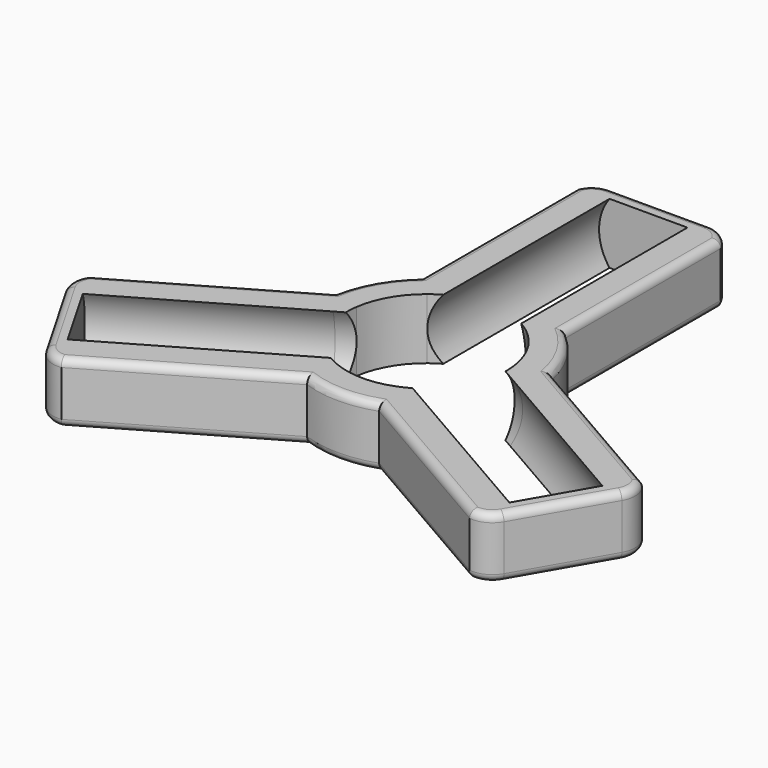
from build123d import *

# Parameters (mm, degrees)
F1_DEPTH       = 4
F3_R           = 6.5
F6_R           = 6.5
F9_R           = 6.5
F11_DEPTH      = 4
F12_T1_DEPTH   = 13
F12_T3_DEPTH   = 13
F12_T5_DEPTH   = 13
F12_T10_DEPTH  = 30.5455488499
F12_S11_R      = 14.5
F12_T12_DEPTH  = 17
F12_T16_DEPTH  = 30.5455488499
F12_S17_R      = 14.5
F12_T18_DEPTH  = 17
F12_T22_ANGLE  = 57.8931407827
F12_T28_DEPTH  = 30.5455488499
F12_S29_R      = 14.5
F12_T30_DEPTH  = 17
F12_T34_DEPTH  = 30.5455488499
F12_S35_R      = 14.5
F12_T36_DEPTH  = 17
F12_T40_ANGLE  = 57.8931407827
F12_T46_DEPTH  = 30.5455488499
F12_S47_R      = 14.5
F12_T48_DEPTH  = 17
F12_T52_DEPTH  = 30.5455488499
F12_S53_R      = 14.5
F12_T54_DEPTH  = 17
F12_T58_ANGLE  = 57.8931407827
F12_T64_DEPTH  = 30.5455488499
F12_S65_R      = 14.5
F12_T66_DEPTH  = 17
F12_T70_ANGLE  = 57.8931407827
F12_T76_DEPTH  = 30.5455488499
F12_S77_R      = 14.5
F12_T78_DEPTH  = 17
F12_T82_DEPTH  = 30.5455488499
F12_S83_R      = 14.5
F12_T84_DEPTH  = 17
F12_T88_ANGLE  = 57.8931407827
F12_T94_DEPTH  = 30.5455488499
F12_S95_R      = 14.5
F12_T96_DEPTH  = 17
F12_T100_DEPTH = 30.5455488499
F12_S101_R     = 14.5
F12_T102_DEPTH = 17
F12_T106_ANGLE = 57.8931407827
F12_T112_DEPTH = 30.5455488499
F12_S113_R     = 14.5
F12_T114_DEPTH = 17
F12_T116_ANGLE = 111.4637339609
F12_T118_ANGLE = 111.4637339609
F12_T120_ANGLE = 111.4637339609
F12_T122_ANGLE = 111.4637339609
F12_T124_ANGLE = 111.4637339609
F12_T126_ANGLE = 111.4637339609
F12_T128_ANGLE = 111.4637339609
F12_T130_ANGLE = 111.4637339609
F12_T132_ANGLE = 111.4637339609
F12_T134_ANGLE = 111.4637339609
F12_T136_ANGLE = 111.4637339609
F12_T138_ANGLE = 111.4637339609
F12_T143_DEPTH = 30.5455488499
F12_S144_R     = 14.5
F12_T145_DEPTH = 17
F12_T148_ANGLE = 57.8931407827
F12_T155_ANGLE = 57.8931407827
F12_T159_DEPTH = 30.5455488499
F12_S160_R     = 14.5
F12_T161_DEPTH = 17
F12_T167_DEPTH = 30.5455488499
F12_S168_R     = 14.5
F12_T169_DEPTH = 17
F12_T172_ANGLE = 57.8931407827
F12_T179_DEPTH = 30.5455488499
F12_S180_R     = 14.5
F12_T181_DEPTH = 17
F12_T184_ANGLE = 57.8931407827
F12_T191_ANGLE = 57.8931407827
F12_T195_DEPTH = 30.5455488499
F12_S196_R     = 14.5
F12_T197_DEPTH = 17
F12_T203_DEPTH = 30.5455488499
F12_S204_R     = 14.5
F12_T205_DEPTH = 17
F12_T208_ANGLE = 57.8931407827
F12_T215_ANGLE = 57.8931407827
F12_T219_DEPTH = 30.5455488499
F12_S220_R     = 14.5
F12_T221_DEPTH = 17
F12_T227_DEPTH = 30.5455488499
F12_S228_R     = 14.5
F12_T229_DEPTH = 17
F12_T232_ANGLE = 57.8931407827
F12_T239_ANGLE = 57.8931407827
F12_T243_DEPTH = 30.5455488499
F12_S244_R     = 14.5
F12_T245_DEPTH = 17
F12_T251_DEPTH = 30.5455488499
F12_S252_R     = 14.5
F12_T253_DEPTH = 17
F12_T256_ANGLE = 57.8931407827
F12_T263_ANGLE = 57.8931407827
F12_T267_DEPTH = 30.5455488499
F12_S268_R     = 14.5
F12_T269_DEPTH = 17
F12_T275_DEPTH = 30.5455488499
F12_S276_R     = 14.5
F12_T277_DEPTH = 17
F12_T280_ANGLE = 57.8931407827


# Not quite as in the source:
# - a fillet or chamfer that OpenCascade refuses, or shapes differently, is made with other operations: its cross-section is extruded or revolved along the edge and cut away or added


with BuildPart() as f1:
    # F0 (on Top) → F1 (new body, symmetric)
    with BuildSketch(Plane.XY):
        with BuildLine():
            ThreePointArc((-9.5, 10.9544511501), (-8.0626945002, 12.0516786133), (-6.5, 12.9614813968))
            Line((-6.5, 12.9614813968), (-6.5, 36.5))
            Line((-6.5, 36.5), (-9.5, 36.5))
            Line((-9.5, 36.5), (-9.5, 10.9544511501))
        make_face()
        with BuildLine():
            Line((6.5, 36.5), (6.5, 12.9614813968))
            ThreePointArc((6.5, 12.9614813968), (8.0626945002, 12.0516786133), (9.5, 10.9544511501))
            Line((9.5, 10.9544511501), (9.5, 36.5))
            Line((9.5, 36.5), (6.5, 36.5))
        make_face()
        with BuildLine():
            ThreePointArc((0, 10.5), (3.4398242587, 9.9205649571), (6.5, 8.2462112512))
            Line((6.5, 8.2462112512), (6.5, 12.9614813968))
            ThreePointArc((6.5, 12.9614813968), (3.3397993762, 14.1101289904), (0, 14.5))
            Line((0, 14.5), (0, 10.5))
        make_face()
        with BuildLine():
            ThreePointArc((6.5, 8.2462112512), (9.0932667397, 5.25), (10.3914284285, 1.506059499))
            Line((10.3914284285, 1.506059499), (14.4749721603, -0.8515755738))
            ThreePointArc((14.4749721603, -0.8515755738), (14.4937416895, -0.4259716395), (14.5, 0))
            ThreePointArc((14.5, 0), (14.4340583035, 1.3812895755), (14.2368329805, 2.7500157609))
            ThreePointArc((14.2368329805, 2.7500157609), (12.5573683549, 7.25), (9.5, 10.9544511501))
            ThreePointArc((9.5, 10.9544511501), (8.0626945002, 12.0516786133), (6.5, 12.9614813968))
            Line((6.5, 12.9614813968), (6.5, 8.2462112512))
        make_face()
        with BuildLine():
            ThreePointArc((-6.5, 8.2462112512), (-3.4398242587, 9.9205649571), (0, 10.5))
            Line((0, 10.5), (0, 14.5))
            ThreePointArc((0, 14.5), (-3.3397993762, 14.1101289904), (-6.5, 12.9614813968))
            Line((-6.5, 12.9614813968), (-6.5, 8.2462112512))
        make_face()
        with BuildLine():
            ThreePointArc((-10.3914284285, 1.506059499), (-9.0932667397, 5.25), (-6.5, 8.2462112512))
            Line((-6.5, 8.2462112512), (-6.5, 12.9614813968))
            ThreePointArc((-6.5, 12.9614813968), (-8.0626945002, 12.0516786133), (-9.5, 10.9544511501))
            ThreePointArc((-9.5, 10.9544511501), (-12.5573683549, 7.25), (-14.2368329805, 2.7500157609))
            ThreePointArc((-14.2368329805, 2.7500157609), (-14.4684070874, 0.9566589535), (-14.4749721603, -0.8515755738))
            Line((-14.4749721603, -0.8515755738), (-10.3914284285, 1.506059499))
        make_face()
        with BuildLine():
            Line((-34.8599272381, -12.6208348754), (-14.4749721603, -0.8515755738))
            ThreePointArc((-14.4749721603, -0.8515755738), (-14.4684070874, 0.9566589535), (-14.2368329805, 2.7500157609))
            Line((-14.2368329805, 2.7500157609), (-36.3599272381, -10.022758664))
            Line((-36.3599272381, -10.022758664), (-34.8599272381, -12.6208348754))
        make_face()
        with BuildLine():
            Line((-12.5573683549, -7.25), (-9.0932667397, -5.25))
            ThreePointArc((-9.0932667397, -5.25), (-10.3113734022, -1.981307286), (-10.3914284285, 1.506059499))
            Line((-10.3914284285, 1.506059499), (-14.4749721603, -0.8515755738))
            ThreePointArc((-14.4749721603, -0.8515755738), (-13.8896298445, -4.1627133919), (-12.5573683549, -7.25))
        make_face()
        with BuildLine():
            Line((-7.9749721603, -12.109905823), (-3.8914284285, -9.7522707502))
            ThreePointArc((-3.8914284285, -9.7522707502), (-6.8715491434, -7.9392576712), (-9.0932667397, -5.25))
            Line((-9.0932667397, -5.25), (-12.5573683549, -7.25))
            ThreePointArc((-12.5573683549, -7.25), (-10.5498304683, -9.9474155985), (-7.9749721603, -12.109905823))
        make_face()
        with BuildLine():
            ThreePointArc((-4.7368329805, -13.704466911), (-6.4057125872, -13.0083375667), (-7.9749721603, -12.109905823))
            Line((-7.9749721603, -12.109905823), (-28.3599272381, -23.8791651246))
            Line((-28.3599272381, -23.8791651246), (-26.8599272381, -26.477241336))
            Line((-26.8599272381, -26.477241336), (-4.7368329805, -13.704466911))
        make_face()
        with BuildLine():
            Line((7.9749721603, -12.109905823), (3.8914284285, -9.7522707502))
            ThreePointArc((3.8914284285, -9.7522707502), (0, -10.5), (-3.8914284285, -9.7522707502))
            Line((-3.8914284285, -9.7522707502), (-7.9749721603, -12.109905823))
            ThreePointArc((-7.9749721603, -12.109905823), (-6.4057125872, -13.0083375667), (-4.7368329805, -13.704466911))
            ThreePointArc((-4.7368329805, -13.704466911), (0, -14.5), (4.7368329805, -13.704466911))
            ThreePointArc((4.7368329805, -13.704466911), (6.4057125872, -13.0083375667), (7.9749721603, -12.109905823))
        make_face()
        with BuildLine():
            Line((28.3599272381, -23.8791651246), (7.9749721603, -12.109905823))
            ThreePointArc((7.9749721603, -12.109905823), (6.4057125872, -13.0083375667), (4.7368329805, -13.704466911))
            Line((4.7368329805, -13.704466911), (26.8599272381, -26.477241336))
            Line((26.8599272381, -26.477241336), (28.3599272381, -23.8791651246))
        make_face()
        with BuildLine():
            Line((12.5573683549, -7.25), (9.0932667397, -5.25))
            ThreePointArc((9.0932667397, -5.25), (6.8715491434, -7.9392576712), (3.8914284285, -9.7522707502))
            Line((3.8914284285, -9.7522707502), (7.9749721603, -12.109905823))
            ThreePointArc((7.9749721603, -12.109905823), (10.5498304683, -9.9474155985), (12.5573683549, -7.25))
        make_face()
        with BuildLine():
            ThreePointArc((10.3914284285, 1.506059499), (10.4728219335, 0.7549839403), (10.5, 0))
            ThreePointArc((10.5, 0), (10.142221176, -2.7175999736), (9.0932667397, -5.25))
            Line((9.0932667397, -5.25), (12.5573683549, -7.25))
            ThreePointArc((12.5573683549, -7.25), (13.8896298445, -4.1627133919), (14.4749721603, -0.8515755738))
            Line((14.4749721603, -0.8515755738), (10.3914284285, 1.506059499))
        make_face()
        with BuildLine():
            ThreePointArc((14.5, 0), (14.4937416895, -0.4259716395), (14.4749721603, -0.8515755738))
            Line((14.4749721603, -0.8515755738), (34.8599272381, -12.6208348754))
            Line((34.8599272381, -12.6208348754), (36.3599272381, -10.022758664))
            Line((36.3599272381, -10.022758664), (14.2368329805, 2.7500157609))
            ThreePointArc((14.2368329805, 2.7500157609), (14.4340583035, 1.3812895755), (14.5, 0))
        make_face()
        with BuildLine():
            ThreePointArc((0, 14.5), (3.3397993762, 14.1101289904), (6.5, 12.9614813968))
            Line((6.5, 12.9614813968), (6.5, 36.5))
            Line((6.5, 36.5), (0, 36.5))
            Line((0, 36.5), (0, 14.5))
        make_face()
        with BuildLine():
            ThreePointArc((-6.5, 12.9614813968), (-3.3397993762, 14.1101289904), (0, 14.5))
            Line((0, 14.5), (0, 36.5))
            Line((0, 36.5), (-6.5, 36.5))
            Line((-6.5, 36.5), (-6.5, 12.9614813968))
        make_face()
        with BuildLine():
            Line((-31.6099272381, -18.25), (-12.5573683549, -7.25))
            ThreePointArc((-12.5573683549, -7.25), (-13.8896298445, -4.1627133919), (-14.4749721603, -0.8515755738))
            Line((-14.4749721603, -0.8515755738), (-34.8599272381, -12.6208348754))
            Line((-34.8599272381, -12.6208348754), (-31.6099272381, -18.25))
        make_face()
        with BuildLine():
            Line((-28.3599272381, -23.8791651246), (-7.9749721603, -12.109905823))
            ThreePointArc((-7.9749721603, -12.109905823), (-10.5498304683, -9.9474155985), (-12.5573683549, -7.25))
            Line((-12.5573683549, -7.25), (-31.6099272381, -18.25))
            Line((-31.6099272381, -18.25), (-28.3599272381, -23.8791651246))
        make_face()
        with BuildLine():
            Line((31.6099272381, -18.25), (12.5573683549, -7.25))
            ThreePointArc((12.5573683549, -7.25), (10.5498304683, -9.9474155985), (7.9749721603, -12.109905823))
            Line((7.9749721603, -12.109905823), (28.3599272381, -23.8791651246))
            Line((28.3599272381, -23.8791651246), (31.6099272381, -18.25))
        make_face()
        with BuildLine():
            Line((34.8599272381, -12.6208348754), (14.4749721603, -0.8515755738))
            ThreePointArc((14.4749721603, -0.8515755738), (13.8896298445, -4.1627133919), (12.5573683549, -7.25))
            Line((12.5573683549, -7.25), (31.6099272381, -18.25))
            Line((31.6099272381, -18.25), (34.8599272381, -12.6208348754))
        make_face()
    extrude(amount=F1_DEPTH, both=True)

    # F4: sweep along a path in F0
    with BuildLine(Plane.XY) as f4_path:
        Line((0, 36.5), (0, 10.5))
        Line((0, 10.5), (0, 5.0456705503))
    # F3 (on offset) → F4 (sweep, cut)
    with BuildSketch(Plane(origin=(0, 36.5, 0), x_dir=(-1, 0, 0), z_dir=(0, 1, 0))):
        Circle(F3_R)
    sweep(path=f4_path.line, mode=Mode.SUBTRACT)

    # F7: sweep along a path in F0
    with BuildLine(Plane.XY) as f7_path:
        Line((-31.6099272381, -18.25), (-9.0932667397, -5.25))
        Line((-9.0932667397, -5.25), (-4.3696788757, -2.5228352752))
    # F6 (on offset) → F7 (sweep, cut)
    with BuildSketch(Plane(origin=(-31.6099272381, -18.25, 0), x_dir=(0.5, -0.8660254038, 0), z_dir=(-0.8660254038, -0.5, 0))):
        Circle(F6_R)
    sweep(path=f7_path.line, mode=Mode.SUBTRACT)

    # F10: sweep along a path in F0
    with BuildLine(Plane.XY) as f10_path:
        Line((31.6099272381, -18.25), (9.0932667397, -5.25))
        Line((9.0932667397, -5.25), (4.3696788757, -2.5228352752))
    # F9 (on offset) → F10 (sweep, cut)
    with BuildSketch(Plane(origin=(31.6099272381, -18.25, 0), x_dir=(0.5, 0.8660254038, 0), z_dir=(0.8660254038, -0.5, 0))):
        Circle(F9_R)
    sweep(path=f10_path.line, mode=Mode.SUBTRACT)

    # F0 (on Top) → F11 (join, symmetric)
    with BuildSketch(Plane.XY):
        with BuildLine():
            Line((0, 36.5), (6.5, 36.5))
            Line((6.5, 36.5), (9.5, 36.5))
            ThreePointArc((9.5, 36.5), (8.3027756377, 37.9541634566), (6.5, 38.5))
            Line((6.5, 38.5), (0, 38.5))
            Line((0, 38.5), (-6.5, 38.5))
            ThreePointArc((-6.5, 38.5), (-8.3027756377, 37.9541634566), (-9.5, 36.5))
            Line((-9.5, 36.5), (-6.5, 36.5))
            Line((-6.5, 36.5), (0, 36.5))
        make_face()
        with BuildLine():
            Line((-26.8599272381, -26.477241336), (-28.3599272381, -23.8791651246))
            Line((-28.3599272381, -23.8791651246), (-31.6099272381, -18.25))
            Line((-31.6099272381, -18.25), (-34.8599272381, -12.6208348754))
            Line((-34.8599272381, -12.6208348754), (-36.3599272381, -10.022758664))
            ThreePointArc((-36.3599272381, -10.022758664), (-37.0206575517, -11.7866671041), (-36.5919780457, -13.6208348754))
            Line((-36.5919780457, -13.6208348754), (-33.3419780457, -19.25))
            Line((-33.3419780457, -19.25), (-30.0919780457, -24.8791651246))
            ThreePointArc((-30.0919780457, -24.8791651246), (-28.7178819139, -26.1674963525), (-26.8599272381, -26.477241336))
        make_face()
        with BuildLine():
            Line((36.3599272381, -10.022758664), (34.8599272381, -12.6208348754))
            Line((34.8599272381, -12.6208348754), (31.6099272381, -18.25))
            Line((31.6099272381, -18.25), (28.3599272381, -23.8791651246))
            Line((28.3599272381, -23.8791651246), (26.8599272381, -26.477241336))
            ThreePointArc((26.8599272381, -26.477241336), (28.7178819139, -26.1674963525), (30.0919780457, -24.8791651246))
            Line((30.0919780457, -24.8791651246), (33.3419780457, -19.25))
            Line((33.3419780457, -19.25), (36.5919780457, -13.6208348754))
            ThreePointArc((36.5919780457, -13.6208348754), (37.0206575517, -11.7866671041), (36.3599272381, -10.022758664))
        make_face()
    extrude(amount=F11_DEPTH, both=True)

    # F12: fillet of radius 1 on 24 edges, made by hand

    # F12_s2 → F12_t1 (cut)
    with BuildSketch(Plane.YZ.offset(-6.5)):
        with BuildLine():
            ThreePointArc((37.5, -4), (38.2071067812, -3.7071067812), (38.5, -3))
            Line((38.5, -3), (38.5, -4))
            Line((38.5, -4), (37.5, -4))
        make_face()
        with BuildLine():
            ThreePointArc((37.5, 4), (38.2071067812, 3.7071067812), (38.5, 3))
            Line((38.5, 3), (38.5, 4))
            Line((38.5, 4), (37.5, 4))
        make_face()
    extrude(amount=F12_T1_DEPTH, mode=Mode.SUBTRACT)

    # F12_s4 → F12_t3 (cut)
    with BuildSketch(Plane(origin=(-3.25, 5.6291651246, 0), x_dir=(0, 0, 1), z_dir=(0.5, -0.8660254038, 0))):
        with BuildLine():
            ThreePointArc((-4, 37.5), (-3.7071067812, 38.2071067812), (-3, 38.5))
            Line((-3, 38.5), (-4, 38.5))
            Line((-4, 38.5), (-4, 37.5))
        make_face()
        with BuildLine():
            ThreePointArc((4, 37.5), (3.7071067812, 38.2071067812), (3, 38.5))
            Line((3, 38.5), (4, 38.5))
            Line((4, 38.5), (4, 37.5))
        make_face()
    extrude(amount=F12_T3_DEPTH, mode=Mode.SUBTRACT)

    # F12_s6 → F12_t5 (cut)
    with BuildSketch(Plane(origin=(-3.25, -5.6291651246, 0), x_dir=(0, 0, 1), z_dir=(0.5, 0.8660254038, 0))):
        with BuildLine():
            ThreePointArc((-4, 37.5), (-3.7071067812, 38.2071067812), (-3, 38.5))
            Line((-3, 38.5), (-4, 38.5))
            Line((-4, 38.5), (-4, 37.5))
        make_face()
        with BuildLine():
            ThreePointArc((4, 37.5), (3.7071067812, 38.2071067812), (3, 38.5))
            Line((3, 38.5), (4, 38.5))
            Line((4, 38.5), (4, 37.5))
        make_face()
    extrude(amount=F12_T5_DEPTH, mode=Mode.SUBTRACT)


with BuildPart() as f12_tool8:
    # F12_s9 → F12_t10 (new body)
    with BuildSketch(Plane.XZ.offset(-39)):
        with BuildLine():
            ThreePointArc((-9.5, -3), (-9.2071067812, -3.7071067812), (-8.5, -4))
            Line((-8.5, -4), (-9.5, -4))
            Line((-9.5, -4), (-9.5, -3))
        make_face()
    extrude(amount=F12_T10_DEPTH)

    # F12_s11 → F12_t12 (cut, symmetric)
    with BuildSketch(Plane.XY.offset(-3.5)):
        Circle(F12_S11_R)
    extrude(amount=F12_T12_DEPTH, both=True, mode=Mode.SUBTRACT)


with BuildPart() as f1_1:
    add(f1.part)

    # F12_t7: cut F12_tool8
    add(f12_tool8.part, mode=Mode.SUBTRACT)


with BuildPart() as f12_tool14:
    # F12_s15 → F12_t16 (new body)
    with BuildSketch(Plane.XZ.offset(-8.4544511501)):
        with BuildLine():
            ThreePointArc((8.5, -4), (9.2071067812, -3.7071067812), (9.5, -3))
            Line((9.5, -3), (9.5, -4))
            Line((9.5, -4), (8.5, -4))
        make_face()
    extrude(amount=-F12_T16_DEPTH)

    # F12_s17 → F12_t18 (cut, symmetric)
    with BuildSketch(Plane.XY.offset(-3.5)):
        Circle(F12_S17_R)
    extrude(amount=F12_T18_DEPTH, both=True, mode=Mode.SUBTRACT)


with BuildPart() as f1_2:
    add(f1_1.part)

    # F12_t13: cut F12_tool14
    add(f12_tool14.part, mode=Mode.SUBTRACT)


with BuildPart() as f12_tool20:
    # F12_s21 → F12_t22 (revolve)
    with BuildSketch(Plane(origin=(0, 0, 0), x_dir=(0, 0, 1), z_dir=(0.8566866434, 0.5158371787, 0))):
        with BuildLine():
            ThreePointArc((-4, -13.5), (-3.7071067812, -14.2071067812), (-3, -14.5))
            Line((-3, -14.5), (-4, -14.5))
            Line((-4, -14.5), (-4, -13.5))
        make_face()
    revolve(axis=Axis((0, 0, -4), (0, 0, 1)), revolution_arc=F12_T22_ANGLE)

    split(bisect_by=Plane.YZ.offset(-9.5), keep=Keep.BOTTOM)

    split(bisect_by=Plane(origin=(-4.75, 8.227241336, 0), x_dir=(0, 0, 1), z_dir=(-0.5, 0.8660254038, 0)), keep=Keep.TOP)


with BuildPart() as f1_3:
    add(f1_2.part)

    # F12_t19: cut F12_tool20
    add(f12_tool20.part, mode=Mode.SUBTRACT)


with BuildPart() as f12_tool26:
    # F12_s27 → F12_t28 (new body)
    with BuildSketch(Plane(origin=(-7.321769471, -4.2272255751, 0), x_dir=(0, 0, 1), z_dir=(-0.8660254038, -0.5, 0))):
        with BuildLine():
            ThreePointArc((-4, 8.5), (-3.7071067812, 9.2071067812), (-3, 9.5))
            Line((-3, 9.5), (-4, 9.5))
            Line((-4, 9.5), (-4, 8.5))
        make_face()
    extrude(amount=F12_T28_DEPTH)

    # F12_s29 → F12_t30 (cut, symmetric)
    with BuildSketch(Plane.XY.offset(-3.5)):
        Circle(F12_S29_R)
    extrude(amount=F12_T30_DEPTH, both=True, mode=Mode.SUBTRACT)


with BuildPart() as f1_4:
    add(f1_3.part)

    # F12_t25: cut F12_tool26
    add(f12_tool26.part, mode=Mode.SUBTRACT)


with BuildPart() as f12_tool32:
    # F12_s33 → F12_t34 (new body)
    with BuildSketch(Plane(origin=(-33.7749907476, -19.5, 0), x_dir=(0, 0, 1), z_dir=(0.8660254038, 0.5, 0))):
        with BuildLine():
            ThreePointArc((-4, 8.5), (-3.7071067812, 9.2071067812), (-3, 9.5))
            Line((-3, 9.5), (-4, 9.5))
            Line((-4, 9.5), (-4, 8.5))
        make_face()
    extrude(amount=F12_T34_DEPTH)

    # F12_s35 → F12_t36 (cut, symmetric)
    with BuildSketch(Plane.XY.offset(-3.5)):
        Circle(F12_S35_R)
    extrude(amount=F12_T36_DEPTH, both=True, mode=Mode.SUBTRACT)


with BuildPart() as f1_5:
    add(f1_4.part)

    # F12_t31: cut F12_tool32
    add(f12_tool32.part, mode=Mode.SUBTRACT)


with BuildPart() as f12_tool38:
    # F12_s39 → F12_t40 (revolve)
    with BuildSketch(Plane(origin=(0, 0, 0), x_dir=(0, 0, 1), z_dir=(-0.8750714227, 0.4839938069, 0))):
        with BuildLine():
            ThreePointArc((-4, -13.5), (-3.7071067812, -14.2071067812), (-3, -14.5))
            Line((-3, -14.5), (-4, -14.5))
            Line((-4, -14.5), (-4, -13.5))
        make_face()
    revolve(axis=Axis((0, 0, -4), (0, 0, 1)), revolution_arc=F12_T40_ANGLE)

    split(bisect_by=Plane(origin=(-4.75, -8.227241336, 0), x_dir=(0, 0, 1), z_dir=(-0.5, -0.8660254038, 0)), keep=Keep.TOP)

    split(bisect_by=Plane(origin=(4.75, -8.227241336, 0), x_dir=(0, 0, 1), z_dir=(0.5, -0.8660254038, 0)), keep=Keep.TOP)


with BuildPart() as f1_6:
    add(f1_5.part)

    # F12_t37: cut F12_tool38
    add(f12_tool38.part, mode=Mode.SUBTRACT)


with BuildPart() as f12_tool44:
    # F12_s45 → F12_t46 (new body)
    with BuildSketch(Plane(origin=(7.321769471, -4.2272255751, 0), x_dir=(0, 0, 1), z_dir=(0.8660254038, -0.5, 0))):
        with BuildLine():
            ThreePointArc((-4, 8.5), (-3.7071067812, 9.2071067812), (-3, 9.5))
            Line((-3, 9.5), (-4, 9.5))
            Line((-4, 9.5), (-4, 8.5))
        make_face()
    extrude(amount=F12_T46_DEPTH)

    # F12_s47 → F12_t48 (cut, symmetric)
    with BuildSketch(Plane.XY.offset(-3.5)):
        Circle(F12_S47_R)
    extrude(amount=F12_T48_DEPTH, both=True, mode=Mode.SUBTRACT)


with BuildPart() as f1_7:
    add(f1_6.part)

    # F12_t43: cut F12_tool44
    add(f12_tool44.part, mode=Mode.SUBTRACT)


with BuildPart() as f12_tool50:
    # F12_s51 → F12_t52 (new body)
    with BuildSketch(Plane(origin=(33.7749907476, -19.5, 0), x_dir=(0, 0, 1), z_dir=(-0.8660254038, 0.5, 0))):
        with BuildLine():
            ThreePointArc((-4, 8.5), (-3.7071067812, 9.2071067812), (-3, 9.5))
            Line((-3, 9.5), (-4, 9.5))
            Line((-4, 9.5), (-4, 8.5))
        make_face()
    extrude(amount=F12_T52_DEPTH)

    # F12_s53 → F12_t54 (cut, symmetric)
    with BuildSketch(Plane.XY.offset(-3.5)):
        Circle(F12_S53_R)
    extrude(amount=F12_T54_DEPTH, both=True, mode=Mode.SUBTRACT)


with BuildPart() as f1_8:
    add(f1_7.part)

    # F12_t49: cut F12_tool50
    add(f12_tool50.part, mode=Mode.SUBTRACT)


with BuildPart() as f12_tool56:
    # F12_s57 → F12_t58 (revolve)
    with BuildSketch(Plane(origin=(0, 0, 0), x_dir=(0, 0, 1), z_dir=(0.0183847793, -0.9998309857, 0))):
        with BuildLine():
            ThreePointArc((-4, -13.5), (-3.7071067812, -14.2071067812), (-3, -14.5))
            Line((-3, -14.5), (-4, -14.5))
            Line((-4, -14.5), (-4, -13.5))
        make_face()
    revolve(axis=Axis((0, 0, -4), (0, 0, 1)), revolution_arc=F12_T58_ANGLE)

    split(bisect_by=Plane.YZ.offset(9.5), keep=Keep.TOP)

    split(bisect_by=Plane(origin=(4.75, 8.227241336, 0), x_dir=(0, 0, 1), z_dir=(0.5, 0.8660254038, 0)), keep=Keep.TOP)


with BuildPart() as f1_9:
    add(f1_8.part)

    # F12_t55: cut F12_tool56
    add(f12_tool56.part, mode=Mode.SUBTRACT)


with BuildPart() as f12_tool62:
    # F12_s63 → F12_t64 (new body)
    with BuildSketch(Plane.XZ.offset(-8.4544511501)):
        with BuildLine():
            ThreePointArc((8.5, 4), (9.2071067812, 3.7071067812), (9.5, 3))
            Line((9.5, 3), (9.5, 4))
            Line((9.5, 4), (8.5, 4))
        make_face()
    extrude(amount=-F12_T64_DEPTH)

    # F12_s65 → F12_t66 (cut, symmetric)
    with BuildSketch(Plane.XY.offset(3.5)):
        Circle(F12_S65_R)
    extrude(amount=F12_T66_DEPTH, both=True, mode=Mode.SUBTRACT)


with BuildPart() as f1_10:
    add(f1_9.part)

    # F12_t61: cut F12_tool62
    add(f12_tool62.part, mode=Mode.SUBTRACT)


with BuildPart() as f12_tool68:
    # F12_s69 → F12_t70 (revolve)
    with BuildSketch(Plane(origin=(0, 0, 0), x_dir=(0, 0, 1), z_dir=(0.0183847793, -0.9998309857, 0))):
        with BuildLine():
            ThreePointArc((4, -13.5), (3.7071067812, -14.2071067812), (3, -14.5))
            Line((3, -14.5), (4, -14.5))
            Line((4, -14.5), (4, -13.5))
        make_face()
    revolve(axis=Axis((0, 0, 4), (0, 0, 1)), revolution_arc=F12_T70_ANGLE)

    split(bisect_by=Plane.YZ.offset(9.5), keep=Keep.TOP)

    split(bisect_by=Plane(origin=(4.75, 8.227241336, 0), x_dir=(0, 0, 1), z_dir=(0.5, 0.8660254038, 0)), keep=Keep.TOP)


with BuildPart() as f1_11:
    add(f1_10.part)

    # F12_t67: cut F12_tool68
    add(f12_tool68.part, mode=Mode.SUBTRACT)


with BuildPart() as f12_tool74:
    # F12_s75 → F12_t76 (new body)
    with BuildSketch(Plane(origin=(33.7749907476, -19.5, 0), x_dir=(0, 0, 1), z_dir=(-0.8660254038, 0.5, 0))):
        with BuildLine():
            ThreePointArc((4, 8.5), (3.7071067812, 9.2071067812), (3, 9.5))
            Line((3, 9.5), (4, 9.5))
            Line((4, 9.5), (4, 8.5))
        make_face()
    extrude(amount=F12_T76_DEPTH)

    # F12_s77 → F12_t78 (cut, symmetric)
    with BuildSketch(Plane.XY.offset(3.5)):
        Circle(F12_S77_R)
    extrude(amount=F12_T78_DEPTH, both=True, mode=Mode.SUBTRACT)


with BuildPart() as f1_12:
    add(f1_11.part)

    # F12_t73: cut F12_tool74
    add(f12_tool74.part, mode=Mode.SUBTRACT)


with BuildPart() as f12_tool80:
    # F12_s81 → F12_t82 (new body)
    with BuildSketch(Plane(origin=(7.321769471, -4.2272255751, 0), x_dir=(0, 0, 1), z_dir=(0.8660254038, -0.5, 0))):
        with BuildLine():
            ThreePointArc((4, 8.5), (3.7071067812, 9.2071067812), (3, 9.5))
            Line((3, 9.5), (4, 9.5))
            Line((4, 9.5), (4, 8.5))
        make_face()
    extrude(amount=F12_T82_DEPTH)

    # F12_s83 → F12_t84 (cut, symmetric)
    with BuildSketch(Plane.XY.offset(3.5)):
        Circle(F12_S83_R)
    extrude(amount=F12_T84_DEPTH, both=True, mode=Mode.SUBTRACT)


with BuildPart() as f1_13:
    add(f1_12.part)

    # F12_t79: cut F12_tool80
    add(f12_tool80.part, mode=Mode.SUBTRACT)


with BuildPart() as f12_tool86:
    # F12_s87 → F12_t88 (revolve)
    with BuildSketch(Plane(origin=(0, 0, 0), x_dir=(0, 0, 1), z_dir=(-0.8750714227, 0.4839938069, 0))):
        with BuildLine():
            ThreePointArc((4, -13.5), (3.7071067812, -14.2071067812), (3, -14.5))
            Line((3, -14.5), (4, -14.5))
            Line((4, -14.5), (4, -13.5))
        make_face()
    revolve(axis=Axis((0, 0, 4), (0, 0, 1)), revolution_arc=F12_T88_ANGLE)

    split(bisect_by=Plane(origin=(-4.75, -8.227241336, 0), x_dir=(0, 0, 1), z_dir=(-0.5, -0.8660254038, 0)), keep=Keep.TOP)

    split(bisect_by=Plane(origin=(4.75, -8.227241336, 0), x_dir=(0, 0, 1), z_dir=(0.5, -0.8660254038, 0)), keep=Keep.TOP)


with BuildPart() as f1_14:
    add(f1_13.part)

    # F12_t85: cut F12_tool86
    add(f12_tool86.part, mode=Mode.SUBTRACT)


with BuildPart() as f12_tool92:
    # F12_s93 → F12_t94 (new body)
    with BuildSketch(Plane(origin=(-33.7749907476, -19.5, 0), x_dir=(0, 0, 1), z_dir=(0.8660254038, 0.5, 0))):
        with BuildLine():
            ThreePointArc((4, 8.5), (3.7071067812, 9.2071067812), (3, 9.5))
            Line((3, 9.5), (4, 9.5))
            Line((4, 9.5), (4, 8.5))
        make_face()
    extrude(amount=F12_T94_DEPTH)

    # F12_s95 → F12_t96 (cut, symmetric)
    with BuildSketch(Plane.XY.offset(3.5)):
        Circle(F12_S95_R)
    extrude(amount=F12_T96_DEPTH, both=True, mode=Mode.SUBTRACT)


with BuildPart() as f1_15:
    add(f1_14.part)

    # F12_t91: cut F12_tool92
    add(f12_tool92.part, mode=Mode.SUBTRACT)


with BuildPart() as f12_tool98:
    # F12_s99 → F12_t100 (new body)
    with BuildSketch(Plane(origin=(-7.321769471, -4.2272255751, 0), x_dir=(0, 0, 1), z_dir=(-0.8660254038, -0.5, 0))):
        with BuildLine():
            ThreePointArc((4, 8.5), (3.7071067812, 9.2071067812), (3, 9.5))
            Line((3, 9.5), (4, 9.5))
            Line((4, 9.5), (4, 8.5))
        make_face()
    extrude(amount=F12_T100_DEPTH)

    # F12_s101 → F12_t102 (cut, symmetric)
    with BuildSketch(Plane.XY.offset(3.5)):
        Circle(F12_S101_R)
    extrude(amount=F12_T102_DEPTH, both=True, mode=Mode.SUBTRACT)


with BuildPart() as f1_16:
    add(f1_15.part)

    # F12_t97: cut F12_tool98
    add(f12_tool98.part, mode=Mode.SUBTRACT)


with BuildPart() as f12_tool104:
    # F12_s105 → F12_t106 (revolve)
    with BuildSketch(Plane(origin=(0, 0, 0), x_dir=(0, 0, 1), z_dir=(0.8566866434, 0.5158371787, 0))):
        with BuildLine():
            ThreePointArc((3, -14.5), (3.7071067812, -14.2071067812), (4, -13.5))
            Line((4, -13.5), (4, -14.5))
            Line((4, -14.5), (3, -14.5))
        make_face()
    revolve(axis=Axis((0, 0, 4), (0, 0, 1)), revolution_arc=F12_T106_ANGLE)

    split(bisect_by=Plane.YZ.offset(-9.5), keep=Keep.BOTTOM)

    split(bisect_by=Plane(origin=(-4.75, 8.227241336, 0), x_dir=(0, 0, 1), z_dir=(-0.5, 0.8660254038, 0)), keep=Keep.TOP)


with BuildPart() as f1_17:
    add(f1_16.part)

    # F12_t103: cut F12_tool104
    add(f12_tool104.part, mode=Mode.SUBTRACT)


with BuildPart() as f12_tool110:
    # F12_s111 → F12_t112 (new body)
    with BuildSketch(Plane.XZ.offset(-39)):
        with BuildLine():
            ThreePointArc((-9.5, 3), (-9.2071067812, 3.7071067812), (-8.5, 4))
            Line((-8.5, 4), (-9.5, 4))
            Line((-9.5, 4), (-9.5, 3))
        make_face()
    extrude(amount=F12_T112_DEPTH)

    # F12_s113 → F12_t114 (cut, symmetric)
    with BuildSketch(Plane.XY.offset(3.5)):
        Circle(F12_S113_R)
    extrude(amount=F12_T114_DEPTH, both=True, mode=Mode.SUBTRACT)


with BuildPart() as f1_18:
    add(f1_17.part)

    # F12_t109: cut F12_tool110
    add(f12_tool110.part, mode=Mode.SUBTRACT)

    # F12_s115 → F12_t116 (revolve, cut)
    with BuildSketch(Plane(origin=(-34.794056996, -5.2225240045, 0), x_dir=(0, 0, 1), z_dir=(0.9889221075, 0.1484353907, 0))):
        with BuildLine():
            ThreePointArc((4, 4.5991854103), (3.7071067812, 3.8920786291), (3, 3.5991854103))
            Line((3, 3.5991854103), (4, 3.5991854103))
            Line((4, 3.5991854103), (4, 4.5991854103))
        make_face()
    revolve(axis=Axis((-33.7773954834, -11.9958348754, 4), (0, 0, 1)), revolution_arc=F12_T116_ANGLE, mode=Mode.SUBTRACT)

    # F12_s117 → F12_t118 (revolve, cut)
    with BuildSketch(Plane(origin=(3.25, -5.6291651246, 0), x_dir=(0, 0, 1), z_dir=(-0.5, 0.8660254038, 0))):
        with BuildLine():
            ThreePointArc((4, -37.5), (3.7071067812, -38.2071067812), (3, -38.5))
            Line((3, -38.5), (4, -38.5))
            Line((4, -38.5), (4, -37.5))
        make_face()
    revolve(axis=Axis((-27.2773954834, -23.2541651246, 4), (0, 0, 1)), revolution_arc=F12_T118_ANGLE, mode=Mode.SUBTRACT)

    # F12_s119 → F12_t120 (revolve, cut)
    with BuildSketch(Plane(origin=(21.9198669578, -27.5212752569, 0), x_dir=(0, 0, 1), z_dir=(-0.623009873, 0.7822139721, 0))):
        with BuildLine():
            ThreePointArc((4, 4.5991854103), (3.7071067812, 3.8920786291), (3, 3.5991854103))
            Line((3, 3.5991854103), (4, 3.5991854103))
            Line((4, 3.5991854103), (4, 4.5991854103))
        make_face()
    revolve(axis=Axis((27.2773954834, -23.2541651246, 4), (0, 0, 1)), revolution_arc=F12_T120_ANGLE, mode=Mode.SUBTRACT)

    # F12_s121 → F12_t122 (revolve, cut)
    with BuildSketch(Plane(origin=(3.25, 5.6291651246, 0), x_dir=(0, 0, 1), z_dir=(-0.5, -0.8660254038, 0))):
        with BuildLine():
            ThreePointArc((4, -37.5), (3.7071067812, -38.2071067812), (3, -38.5))
            Line((3, -38.5), (4, -38.5))
            Line((4, -38.5), (4, -37.5))
        make_face()
    revolve(axis=Axis((33.7773954834, -11.9958348754, 4), (0, 0, 1)), revolution_arc=F12_T122_ANGLE, mode=Mode.SUBTRACT)

    # F12_s123 → F12_t124 (revolve, cut)
    with BuildSketch(Plane(origin=(12.8741900382, 32.7437992615, 0), x_dir=(0, 0, 1), z_dir=(-0.3659122346, -0.9306493629, 0))):
        with BuildLine():
            ThreePointArc((4, 4.5991854103), (3.7071067812, 3.8920786291), (3, 3.5991854103))
            Line((3, 3.5991854103), (4, 3.5991854103))
            Line((4, 3.5991854103), (4, 4.5991854103))
        make_face()
    revolve(axis=Axis((6.5, 35.25, 4), (0, 0, 1)), revolution_arc=F12_T124_ANGLE, mode=Mode.SUBTRACT)

    # F12_s125 → F12_t126 (revolve, cut)
    with BuildSketch(Plane.YZ.offset(-6.5)):
        with BuildLine():
            ThreePointArc((37.5, 4), (38.2071067812, 3.7071067812), (38.5, 3))
            Line((38.5, 3), (38.5, 4))
            Line((38.5, 4), (37.5, 4))
        make_face()
    revolve(axis=Axis((-6.5, 35.25, 4), (0, 0, 1)), revolution_arc=F12_T126_ANGLE, mode=Mode.SUBTRACT)

    # F12_s127 → F12_t128 (revolve, cut)
    with BuildSketch(Plane(origin=(21.9198669578, -27.5212752569, 0), x_dir=(0, 0, 1), z_dir=(-0.623009873, 0.7822139721, 0))):
        with BuildLine():
            ThreePointArc((-4, 4.5991854103), (-3.7071067812, 3.8920786291), (-3, 3.5991854103))
            Line((-3, 3.5991854103), (-4, 3.5991854103))
            Line((-4, 3.5991854103), (-4, 4.5991854103))
        make_face()
    revolve(axis=Axis((27.2773954834, -23.2541651246, -4), (0, 0, 1)), revolution_arc=F12_T128_ANGLE, mode=Mode.SUBTRACT)

    # F12_s129 → F12_t130 (revolve, cut)
    with BuildSketch(Plane(origin=(3.25, 5.6291651246, 0), x_dir=(0, 0, 1), z_dir=(-0.5, -0.8660254038, 0))):
        with BuildLine():
            ThreePointArc((-4, -37.5), (-3.7071067812, -38.2071067812), (-3, -38.5))
            Line((-3, -38.5), (-4, -38.5))
            Line((-4, -38.5), (-4, -37.5))
        make_face()
    revolve(axis=Axis((33.7773954834, -11.9958348754, -4), (0, 0, 1)), revolution_arc=F12_T130_ANGLE, mode=Mode.SUBTRACT)

    # F12_s131 → F12_t132 (revolve, cut)
    with BuildSketch(Plane(origin=(-34.794056996, -5.2225240045, 0), x_dir=(0, 0, 1), z_dir=(0.9889221075, 0.1484353907, 0))):
        with BuildLine():
            ThreePointArc((-4, 4.5991854103), (-3.7071067812, 3.8920786291), (-3, 3.5991854103))
            Line((-3, 3.5991854103), (-4, 3.5991854103))
            Line((-4, 3.5991854103), (-4, 4.5991854103))
        make_face()
    revolve(axis=Axis((-33.7773954834, -11.9958348754, -4), (0, 0, 1)), revolution_arc=F12_T132_ANGLE, mode=Mode.SUBTRACT)

    # F12_s133 → F12_t134 (revolve, cut)
    with BuildSketch(Plane(origin=(3.25, -5.6291651246, 0), x_dir=(0, 0, 1), z_dir=(-0.5, 0.8660254038, 0))):
        with BuildLine():
            ThreePointArc((-4, -37.5), (-3.7071067812, -38.2071067812), (-3, -38.5))
            Line((-3, -38.5), (-4, -38.5))
            Line((-4, -38.5), (-4, -37.5))
        make_face()
    revolve(axis=Axis((-27.2773954834, -23.2541651246, -4), (0, 0, 1)), revolution_arc=F12_T134_ANGLE, mode=Mode.SUBTRACT)

    # F12_s135 → F12_t136 (revolve, cut)
    with BuildSketch(Plane(origin=(12.8741900382, 32.7437992615, 0), x_dir=(0, 0, 1), z_dir=(-0.3659122346, -0.9306493629, 0))):
        with BuildLine():
            ThreePointArc((-4, 4.5991854103), (-3.7071067812, 3.8920786291), (-3, 3.5991854103))
            Line((-3, 3.5991854103), (-4, 3.5991854103))
            Line((-4, 3.5991854103), (-4, 4.5991854103))
        make_face()
    revolve(axis=Axis((6.5, 35.25, -4), (0, 0, 1)), revolution_arc=F12_T136_ANGLE, mode=Mode.SUBTRACT)

    # F12_s137 → F12_t138 (revolve, cut)
    with BuildSketch(Plane.YZ.offset(-6.5)):
        with BuildLine():
            ThreePointArc((37.5, -4), (38.2071067812, -3.7071067812), (38.5, -3))
            Line((38.5, -3), (38.5, -4))
            Line((38.5, -4), (37.5, -4))
        make_face()
    revolve(axis=Axis((-6.5, 35.25, -4), (0, 0, 1)), revolution_arc=F12_T138_ANGLE, mode=Mode.SUBTRACT)


with BuildPart() as f12_tool141:
    # F12_s142 → F12_t143 (new body)
    with BuildSketch(Plane.XZ.offset(-39)):
        with BuildLine():
            ThreePointArc((-9.5, -3), (-9.2071067812, -3.7071067812), (-8.5, -4))
            Line((-8.5, -4), (-9.5, -4))
            Line((-9.5, -4), (-9.5, -3))
        make_face()
    extrude(amount=F12_T143_DEPTH)

    # F12_s144 → F12_t145 (intersect, symmetric)
    with BuildSketch(Plane.XY.offset(-3.5)):
        Circle(F12_S144_R)
    extrude(amount=F12_T145_DEPTH, both=True, mode=Mode.INTERSECT)


with BuildPart() as f12_tool146:
    # F12_s147 → F12_t148 (revolve)
    with BuildSketch(Plane(origin=(0, 0, 0), x_dir=(0, 0, 1), z_dir=(0.8566866434, 0.5158371787, 0))):
        with BuildLine():
            ThreePointArc((-4, -13.5), (-3.7071067812, -14.2071067812), (-3, -14.5))
            Line((-3, -14.5), (-4, -14.5))
            Line((-4, -14.5), (-4, -13.5))
        make_face()
    revolve(axis=Axis((0, 0, -4), (0, 0, 1)), revolution_arc=F12_T148_ANGLE)

    split(bisect_by=Plane.YZ.offset(-9.5), keep=Keep.TOP)


with BuildPart() as f12_tool141_1:
    add(f12_tool141.part)

    # F12_t150: intersect F12_tool146
    add(f12_tool146.part, mode=Mode.INTERSECT)


with BuildPart() as f1_19:
    add(f1_18.part)

    # F12_t139: cut F12_tool141
    add(f12_tool141_1.part, mode=Mode.SUBTRACT)


with BuildPart() as f12_tool153:
    # F12_s154 → F12_t155 (revolve)
    with BuildSketch(Plane(origin=(0, 0, 0), x_dir=(0, 0, 1), z_dir=(0.0183847793, -0.9998309857, 0))):
        with BuildLine():
            ThreePointArc((-4, -13.5), (-3.7071067812, -14.2071067812), (-3, -14.5))
            Line((-3, -14.5), (-4, -14.5))
            Line((-4, -14.5), (-4, -13.5))
        make_face()
    revolve(axis=Axis((0, 0, -4), (0, 0, 1)), revolution_arc=F12_T155_ANGLE)

    split(bisect_by=Plane.YZ.offset(9.5), keep=Keep.BOTTOM)


with BuildPart() as f12_tool157:
    # F12_s158 → F12_t159 (new body)
    with BuildSketch(Plane.XZ.offset(-8.4544511501)):
        with BuildLine():
            ThreePointArc((8.5, -4), (9.2071067812, -3.7071067812), (9.5, -3))
            Line((9.5, -3), (9.5, -4))
            Line((9.5, -4), (8.5, -4))
        make_face()
    extrude(amount=-F12_T159_DEPTH)

    # F12_s160 → F12_t161 (intersect, symmetric)
    with BuildSketch(Plane.XY.offset(-3.5)):
        Circle(F12_S160_R)
    extrude(amount=F12_T161_DEPTH, both=True, mode=Mode.INTERSECT)


with BuildPart() as f12_tool153_1:
    add(f12_tool153.part)

    # F12_t162: intersect F12_tool157
    add(f12_tool157.part, mode=Mode.INTERSECT)


with BuildPart() as f1_20:
    add(f1_19.part)

    # F12_t151: cut F12_tool153
    add(f12_tool153_1.part, mode=Mode.SUBTRACT)


with BuildPart() as f12_tool165:
    # F12_s166 → F12_t167 (new body)
    with BuildSketch(Plane(origin=(-7.321769471, -4.2272255751, 0), x_dir=(0, 0, 1), z_dir=(-0.8660254038, -0.5, 0))):
        with BuildLine():
            ThreePointArc((-4, 8.5), (-3.7071067812, 9.2071067812), (-3, 9.5))
            Line((-3, 9.5), (-4, 9.5))
            Line((-4, 9.5), (-4, 8.5))
        make_face()
    extrude(amount=F12_T167_DEPTH)

    # F12_s168 → F12_t169 (intersect, symmetric)
    with BuildSketch(Plane.XY.offset(-3.5)):
        Circle(F12_S168_R)
    extrude(amount=F12_T169_DEPTH, both=True, mode=Mode.INTERSECT)


with BuildPart() as f12_tool170:
    # F12_s171 → F12_t172 (revolve)
    with BuildSketch(Plane(origin=(0, 0, 0), x_dir=(0, 0, 1), z_dir=(0.8566866434, 0.5158371787, 0))):
        with BuildLine():
            ThreePointArc((-4, -13.5), (-3.7071067812, -14.2071067812), (-3, -14.5))
            Line((-3, -14.5), (-4, -14.5))
            Line((-4, -14.5), (-4, -13.5))
        make_face()
    revolve(axis=Axis((0, 0, -4), (0, 0, 1)), revolution_arc=F12_T172_ANGLE)

    split(bisect_by=Plane(origin=(-4.75, 8.227241336, 0), x_dir=(0, 0, 1), z_dir=(0.5, -0.8660254038, 0)), keep=Keep.TOP)


with BuildPart() as f12_tool165_1:
    add(f12_tool165.part)

    # F12_t174: intersect F12_tool170
    add(f12_tool170.part, mode=Mode.INTERSECT)


with BuildPart() as f1_21:
    add(f1_20.part)

    # F12_t163: cut F12_tool165
    add(f12_tool165_1.part, mode=Mode.SUBTRACT)


with BuildPart() as f12_tool177:
    # F12_s178 → F12_t179 (new body)
    with BuildSketch(Plane(origin=(-33.7749907476, -19.5, 0), x_dir=(0, 0, 1), z_dir=(0.8660254038, 0.5, 0))):
        with BuildLine():
            ThreePointArc((-4, 8.5), (-3.7071067812, 9.2071067812), (-3, 9.5))
            Line((-3, 9.5), (-4, 9.5))
            Line((-4, 9.5), (-4, 8.5))
        make_face()
    extrude(amount=F12_T179_DEPTH)

    # F12_s180 → F12_t181 (intersect, symmetric)
    with BuildSketch(Plane.XY.offset(-3.5)):
        Circle(F12_S180_R)
    extrude(amount=F12_T181_DEPTH, both=True, mode=Mode.INTERSECT)


with BuildPart() as f12_tool182:
    # F12_s183 → F12_t184 (revolve)
    with BuildSketch(Plane(origin=(0, 0, 0), x_dir=(0, 0, 1), z_dir=(-0.8750714227, 0.4839938069, 0))):
        with BuildLine():
            ThreePointArc((-4, -13.5), (-3.7071067812, -14.2071067812), (-3, -14.5))
            Line((-3, -14.5), (-4, -14.5))
            Line((-4, -14.5), (-4, -13.5))
        make_face()
    revolve(axis=Axis((0, 0, -4), (0, 0, 1)), revolution_arc=F12_T184_ANGLE)

    split(bisect_by=Plane(origin=(4.75, -8.227241336, 0), x_dir=(0, 0, 1), z_dir=(-0.5, 0.8660254038, 0)), keep=Keep.TOP)


with BuildPart() as f12_tool177_1:
    add(f12_tool177.part)

    # F12_t186: intersect F12_tool182
    add(f12_tool182.part, mode=Mode.INTERSECT)


with BuildPart() as f1_22:
    add(f1_21.part)

    # F12_t175: cut F12_tool177
    add(f12_tool177_1.part, mode=Mode.SUBTRACT)


with BuildPart() as f12_tool189:
    # F12_s190 → F12_t191 (revolve)
    with BuildSketch(Plane(origin=(0, 0, 0), x_dir=(0, 0, 1), z_dir=(-0.8750714227, 0.4839938069, 0))):
        with BuildLine():
            ThreePointArc((-4, -13.5), (-3.7071067812, -14.2071067812), (-3, -14.5))
            Line((-3, -14.5), (-4, -14.5))
            Line((-4, -14.5), (-4, -13.5))
        make_face()
    revolve(axis=Axis((0, 0, -4), (0, 0, 1)), revolution_arc=F12_T191_ANGLE)

    split(bisect_by=Plane(origin=(-4.75, -8.227241336, 0), x_dir=(0, 0, 1), z_dir=(0.5, 0.8660254038, 0)), keep=Keep.TOP)


with BuildPart() as f12_tool193:
    # F12_s194 → F12_t195 (new body)
    with BuildSketch(Plane(origin=(7.321769471, -4.2272255751, 0), x_dir=(0, 0, 1), z_dir=(0.8660254038, -0.5, 0))):
        with BuildLine():
            ThreePointArc((-4, 8.5), (-3.7071067812, 9.2071067812), (-3, 9.5))
            Line((-3, 9.5), (-4, 9.5))
            Line((-4, 9.5), (-4, 8.5))
        make_face()
    extrude(amount=F12_T195_DEPTH)

    # F12_s196 → F12_t197 (intersect, symmetric)
    with BuildSketch(Plane.XY.offset(-3.5)):
        Circle(F12_S196_R)
    extrude(amount=F12_T197_DEPTH, both=True, mode=Mode.INTERSECT)


with BuildPart() as f12_tool189_1:
    add(f12_tool189.part)

    # F12_t198: intersect F12_tool193
    add(f12_tool193.part, mode=Mode.INTERSECT)


with BuildPart() as f1_23:
    add(f1_22.part)

    # F12_t187: cut F12_tool189
    add(f12_tool189_1.part, mode=Mode.SUBTRACT)


with BuildPart() as f12_tool201:
    # F12_s202 → F12_t203 (new body)
    with BuildSketch(Plane(origin=(33.7749907476, -19.5, 0), x_dir=(0, 0, 1), z_dir=(-0.8660254038, 0.5, 0))):
        with BuildLine():
            ThreePointArc((-4, 8.5), (-3.7071067812, 9.2071067812), (-3, 9.5))
            Line((-3, 9.5), (-4, 9.5))
            Line((-4, 9.5), (-4, 8.5))
        make_face()
    extrude(amount=F12_T203_DEPTH)

    # F12_s204 → F12_t205 (intersect, symmetric)
    with BuildSketch(Plane.XY.offset(-3.5)):
        Circle(F12_S204_R)
    extrude(amount=F12_T205_DEPTH, both=True, mode=Mode.INTERSECT)


with BuildPart() as f12_tool206:
    # F12_s207 → F12_t208 (revolve)
    with BuildSketch(Plane(origin=(0, 0, 0), x_dir=(0, 0, 1), z_dir=(0.0183847793, -0.9998309857, 0))):
        with BuildLine():
            ThreePointArc((-4, -13.5), (-3.7071067812, -14.2071067812), (-3, -14.5))
            Line((-3, -14.5), (-4, -14.5))
            Line((-4, -14.5), (-4, -13.5))
        make_face()
    revolve(axis=Axis((0, 0, -4), (0, 0, 1)), revolution_arc=F12_T208_ANGLE)

    split(bisect_by=Plane(origin=(4.75, 8.227241336, 0), x_dir=(0, 0, 1), z_dir=(-0.5, -0.8660254038, 0)), keep=Keep.TOP)


with BuildPart() as f12_tool201_1:
    add(f12_tool201.part)

    # F12_t210: intersect F12_tool206
    add(f12_tool206.part, mode=Mode.INTERSECT)


with BuildPart() as f1_24:
    add(f1_23.part)

    # F12_t199: cut F12_tool201
    add(f12_tool201_1.part, mode=Mode.SUBTRACT)


with BuildPart() as f12_tool213:
    # F12_s214 → F12_t215 (revolve)
    with BuildSketch(Plane(origin=(0, 0, 0), x_dir=(0, 0, 1), z_dir=(0.0183847793, -0.9998309857, 0))):
        with BuildLine():
            ThreePointArc((4, -13.5), (3.7071067812, -14.2071067812), (3, -14.5))
            Line((3, -14.5), (4, -14.5))
            Line((4, -14.5), (4, -13.5))
        make_face()
    revolve(axis=Axis((0, 0, 4), (0, 0, 1)), revolution_arc=F12_T215_ANGLE)

    split(bisect_by=Plane.YZ.offset(9.5), keep=Keep.BOTTOM)


with BuildPart() as f12_tool217:
    # F12_s218 → F12_t219 (new body)
    with BuildSketch(Plane.XZ.offset(-8.4544511501)):
        with BuildLine():
            ThreePointArc((8.5, 4), (9.2071067812, 3.7071067812), (9.5, 3))
            Line((9.5, 3), (9.5, 4))
            Line((9.5, 4), (8.5, 4))
        make_face()
    extrude(amount=-F12_T219_DEPTH)

    # F12_s220 → F12_t221 (intersect, symmetric)
    with BuildSketch(Plane.XY.offset(3.5)):
        Circle(F12_S220_R)
    extrude(amount=F12_T221_DEPTH, both=True, mode=Mode.INTERSECT)


with BuildPart() as f12_tool213_1:
    add(f12_tool213.part)

    # F12_t222: intersect F12_tool217
    add(f12_tool217.part, mode=Mode.INTERSECT)


with BuildPart() as f1_25:
    add(f1_24.part)

    # F12_t211: cut F12_tool213
    add(f12_tool213_1.part, mode=Mode.SUBTRACT)


with BuildPart() as f12_tool225:
    # F12_s226 → F12_t227 (new body)
    with BuildSketch(Plane(origin=(33.7749907476, -19.5, 0), x_dir=(0, 0, 1), z_dir=(-0.8660254038, 0.5, 0))):
        with BuildLine():
            ThreePointArc((4, 8.5), (3.7071067812, 9.2071067812), (3, 9.5))
            Line((3, 9.5), (4, 9.5))
            Line((4, 9.5), (4, 8.5))
        make_face()
    extrude(amount=F12_T227_DEPTH)

    # F12_s228 → F12_t229 (intersect, symmetric)
    with BuildSketch(Plane.XY.offset(3.5)):
        Circle(F12_S228_R)
    extrude(amount=F12_T229_DEPTH, both=True, mode=Mode.INTERSECT)


with BuildPart() as f12_tool230:
    # F12_s231 → F12_t232 (revolve)
    with BuildSketch(Plane(origin=(0, 0, 0), x_dir=(0, 0, 1), z_dir=(0.0183847793, -0.9998309857, 0))):
        with BuildLine():
            ThreePointArc((4, -13.5), (3.7071067812, -14.2071067812), (3, -14.5))
            Line((3, -14.5), (4, -14.5))
            Line((4, -14.5), (4, -13.5))
        make_face()
    revolve(axis=Axis((0, 0, 4), (0, 0, 1)), revolution_arc=F12_T232_ANGLE)

    split(bisect_by=Plane(origin=(4.75, 8.227241336, 0), x_dir=(0, 0, 1), z_dir=(-0.5, -0.8660254038, 0)), keep=Keep.TOP)


with BuildPart() as f12_tool225_1:
    add(f12_tool225.part)

    # F12_t234: intersect F12_tool230
    add(f12_tool230.part, mode=Mode.INTERSECT)


with BuildPart() as f1_26:
    add(f1_25.part)

    # F12_t223: cut F12_tool225
    add(f12_tool225_1.part, mode=Mode.SUBTRACT)


with BuildPart() as f12_tool237:
    # F12_s238 → F12_t239 (revolve)
    with BuildSketch(Plane(origin=(0, 0, 0), x_dir=(0, 0, 1), z_dir=(-0.8750714227, 0.4839938069, 0))):
        with BuildLine():
            ThreePointArc((4, -13.5), (3.7071067812, -14.2071067812), (3, -14.5))
            Line((3, -14.5), (4, -14.5))
            Line((4, -14.5), (4, -13.5))
        make_face()
    revolve(axis=Axis((0, 0, 4), (0, 0, 1)), revolution_arc=F12_T239_ANGLE)

    split(bisect_by=Plane(origin=(-4.75, -8.227241336, 0), x_dir=(0, 0, 1), z_dir=(0.5, 0.8660254038, 0)), keep=Keep.TOP)


with BuildPart() as f12_tool241:
    # F12_s242 → F12_t243 (new body)
    with BuildSketch(Plane(origin=(7.321769471, -4.2272255751, 0), x_dir=(0, 0, 1), z_dir=(0.8660254038, -0.5, 0))):
        with BuildLine():
            ThreePointArc((4, 8.5), (3.7071067812, 9.2071067812), (3, 9.5))
            Line((3, 9.5), (4, 9.5))
            Line((4, 9.5), (4, 8.5))
        make_face()
    extrude(amount=F12_T243_DEPTH)

    # F12_s244 → F12_t245 (intersect, symmetric)
    with BuildSketch(Plane.XY.offset(3.5)):
        Circle(F12_S244_R)
    extrude(amount=F12_T245_DEPTH, both=True, mode=Mode.INTERSECT)


with BuildPart() as f12_tool237_1:
    add(f12_tool237.part)

    # F12_t246: intersect F12_tool241
    add(f12_tool241.part, mode=Mode.INTERSECT)


with BuildPart() as f1_27:
    add(f1_26.part)

    # F12_t235: cut F12_tool237
    add(f12_tool237_1.part, mode=Mode.SUBTRACT)


with BuildPart() as f12_tool249:
    # F12_s250 → F12_t251 (new body)
    with BuildSketch(Plane(origin=(-33.7749907476, -19.5, 0), x_dir=(0, 0, 1), z_dir=(0.8660254038, 0.5, 0))):
        with BuildLine():
            ThreePointArc((4, 8.5), (3.7071067812, 9.2071067812), (3, 9.5))
            Line((3, 9.5), (4, 9.5))
            Line((4, 9.5), (4, 8.5))
        make_face()
    extrude(amount=F12_T251_DEPTH)

    # F12_s252 → F12_t253 (intersect, symmetric)
    with BuildSketch(Plane.XY.offset(3.5)):
        Circle(F12_S252_R)
    extrude(amount=F12_T253_DEPTH, both=True, mode=Mode.INTERSECT)


with BuildPart() as f12_tool254:
    # F12_s255 → F12_t256 (revolve)
    with BuildSketch(Plane(origin=(0, 0, 0), x_dir=(0, 0, 1), z_dir=(-0.8750714227, 0.4839938069, 0))):
        with BuildLine():
            ThreePointArc((4, -13.5), (3.7071067812, -14.2071067812), (3, -14.5))
            Line((3, -14.5), (4, -14.5))
            Line((4, -14.5), (4, -13.5))
        make_face()
    revolve(axis=Axis((0, 0, 4), (0, 0, 1)), revolution_arc=F12_T256_ANGLE)

    split(bisect_by=Plane(origin=(4.75, -8.227241336, 0), x_dir=(0, 0, 1), z_dir=(-0.5, 0.8660254038, 0)), keep=Keep.TOP)


with BuildPart() as f12_tool249_1:
    add(f12_tool249.part)

    # F12_t258: intersect F12_tool254
    add(f12_tool254.part, mode=Mode.INTERSECT)


with BuildPart() as f1_28:
    add(f1_27.part)

    # F12_t247: cut F12_tool249
    add(f12_tool249_1.part, mode=Mode.SUBTRACT)


with BuildPart() as f12_tool261:
    # F12_s262 → F12_t263 (revolve)
    with BuildSketch(Plane(origin=(0, 0, 0), x_dir=(0, 0, 1), z_dir=(0.8566866434, 0.5158371787, 0))):
        with BuildLine():
            ThreePointArc((3, -14.5), (3.7071067812, -14.2071067812), (4, -13.5))
            Line((4, -13.5), (4, -14.5))
            Line((4, -14.5), (3, -14.5))
        make_face()
    revolve(axis=Axis((0, 0, 4), (0, 0, 1)), revolution_arc=F12_T263_ANGLE)

    split(bisect_by=Plane(origin=(-4.75, 8.227241336, 0), x_dir=(0, 0, 1), z_dir=(0.5, -0.8660254038, 0)), keep=Keep.TOP)


with BuildPart() as f12_tool265:
    # F12_s266 → F12_t267 (new body)
    with BuildSketch(Plane(origin=(-7.321769471, -4.2272255751, 0), x_dir=(0, 0, 1), z_dir=(-0.8660254038, -0.5, 0))):
        with BuildLine():
            ThreePointArc((4, 8.5), (3.7071067812, 9.2071067812), (3, 9.5))
            Line((3, 9.5), (4, 9.5))
            Line((4, 9.5), (4, 8.5))
        make_face()
    extrude(amount=F12_T267_DEPTH)

    # F12_s268 → F12_t269 (intersect, symmetric)
    with BuildSketch(Plane.XY.offset(3.5)):
        Circle(F12_S268_R)
    extrude(amount=F12_T269_DEPTH, both=True, mode=Mode.INTERSECT)


with BuildPart() as f12_tool261_1:
    add(f12_tool261.part)

    # F12_t270: intersect F12_tool265
    add(f12_tool265.part, mode=Mode.INTERSECT)


with BuildPart() as f1_29:
    add(f1_28.part)

    # F12_t259: cut F12_tool261
    add(f12_tool261_1.part, mode=Mode.SUBTRACT)


with BuildPart() as f12_tool273:
    # F12_s274 → F12_t275 (new body)
    with BuildSketch(Plane.XZ.offset(-39)):
        with BuildLine():
            ThreePointArc((-9.5, 3), (-9.2071067812, 3.7071067812), (-8.5, 4))
            Line((-8.5, 4), (-9.5, 4))
            Line((-9.5, 4), (-9.5, 3))
        make_face()
    extrude(amount=F12_T275_DEPTH)

    # F12_s276 → F12_t277 (intersect, symmetric)
    with BuildSketch(Plane.XY.offset(3.5)):
        Circle(F12_S276_R)
    extrude(amount=F12_T277_DEPTH, both=True, mode=Mode.INTERSECT)


with BuildPart() as f12_tool278:
    # F12_s279 → F12_t280 (revolve)
    with BuildSketch(Plane(origin=(0, 0, 0), x_dir=(0, 0, 1), z_dir=(0.8566866434, 0.5158371787, 0))):
        with BuildLine():
            ThreePointArc((3, -14.5), (3.7071067812, -14.2071067812), (4, -13.5))
            Line((4, -13.5), (4, -14.5))
            Line((4, -14.5), (3, -14.5))
        make_face()
    revolve(axis=Axis((0, 0, 4), (0, 0, 1)), revolution_arc=F12_T280_ANGLE)

    split(bisect_by=Plane.YZ.offset(-9.5), keep=Keep.TOP)


with BuildPart() as f12_tool273_1:
    add(f12_tool273.part)

    # F12_t282: intersect F12_tool278
    add(f12_tool278.part, mode=Mode.INTERSECT)


with BuildPart() as f1_30:
    add(f1_29.part)

    # F12_t271: cut F12_tool273
    add(f12_tool273_1.part, mode=Mode.SUBTRACT)


solid = f1_30.part
